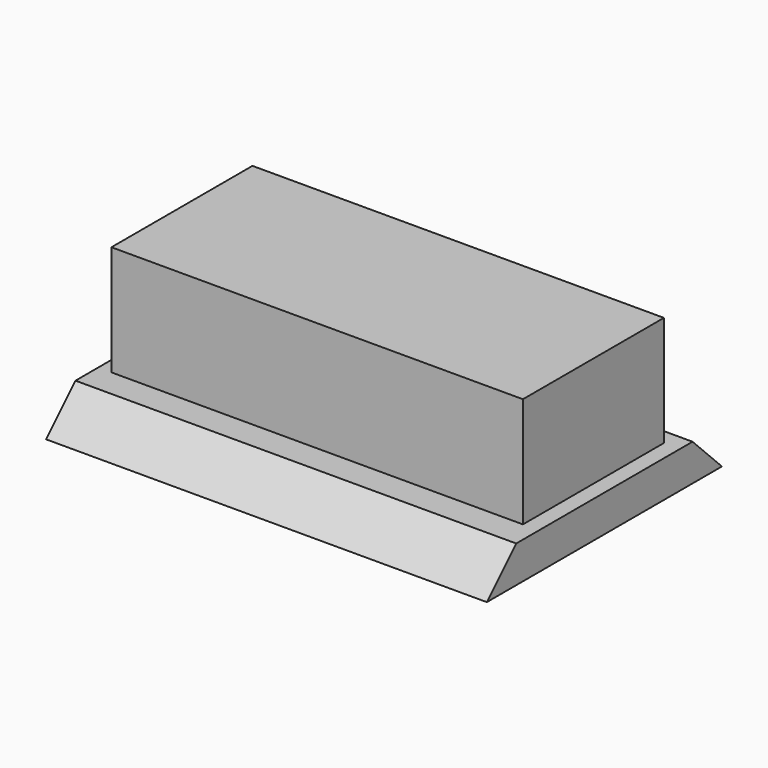
from build123d import *

# Parameters (mm, degrees)
F0_W     = 38.1
F0_H     = 25.4
F1_DEPTH = 3.175
F2_SIZE  = 3.17499
F3_W     = 35.5673587183
F3_H     = 15.2347986586
F4_DEPTH = 9.525


# Not quite as in the source:
# - a fillet or chamfer is up to 0.001 mm smaller than in the source, because OpenCascade refuses the exact size


with BuildPart() as f1:
    # F0 (on Top) → F1 (new body)
    with BuildSketch(Plane.XY):
        with Locations((19.05, -12.7)):
            Rectangle(F0_W, F0_H)
    extrude(amount=F1_DEPTH)

    # F2 (size 3.175 in the source; OpenCascade refuses exactly that, so slightly less here)
    f2_edges = [f1.edges().sort_by_distance(p)[0] for p in [
        (19.05, -25.4, 3.175),
        (19.05, 0, 3.175),
    ]]
    chamfer(f2_edges, length=F2_SIZE)

    # F3 (on face) → F4 (join)
    with BuildSketch(Plane.XY.offset(3.175)):
        with Locations((18.9271715353, -12.1486445423)):
            Rectangle(F3_W, F3_H)
    extrude(amount=F4_DEPTH)


solid = f1.part
